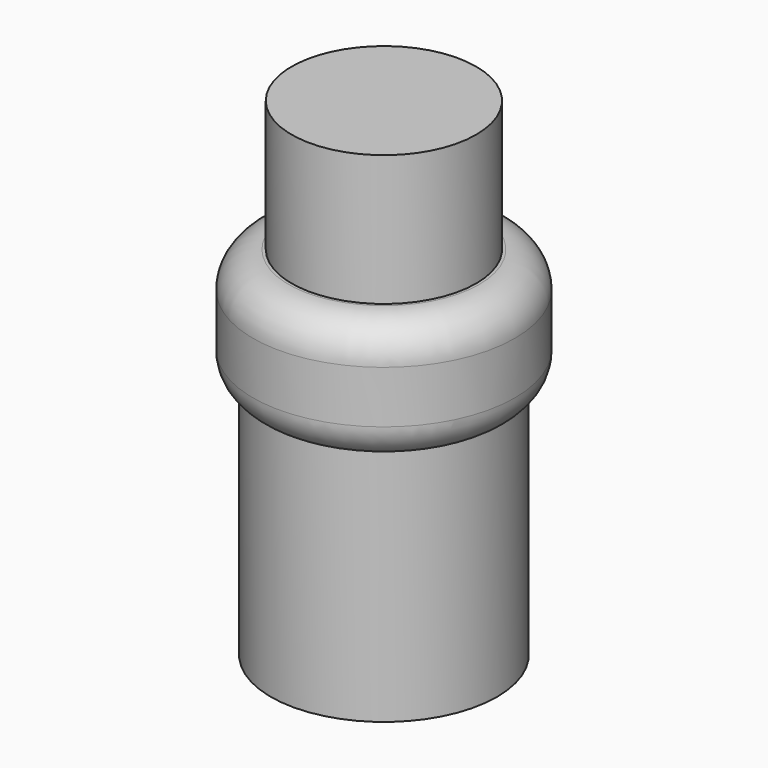
from build123d import *

# Parameters (mm, degrees)
F0_R     = 4.75
F1_DEPTH = 10
F2_R     = 5.5
F3_DEPTH = 5
F4_R     = 3.875
F5_DEPTH = 5.5


# Not quite as in the source:
# - a fillet or chamfer that OpenCascade refuses, or shapes differently, is made with other operations: its cross-section is extruded or revolved along the edge and cut away or added


with BuildPart() as f1:
    # F0 (on Top) → F1 (new body)
    with BuildSketch(Plane.XY):
        Circle(F0_R)
    extrude(amount=F1_DEPTH)

    # F2 (on face) → F3 (join)
    with BuildSketch(Plane.XY.offset(10)):
        Circle(F2_R)
    extrude(amount=F3_DEPTH)

    # F4 (on face) → F5 (join)
    with BuildSketch(Plane.XY.offset(15)):
        Circle(F4_R)
    extrude(amount=F5_DEPTH)

    # F6: fillet of radius 1.5 on 2 edges, made by hand

    # F6_s1 → F6_t2 (revolve, cut)
    with BuildSketch(Plane.XZ):
        with BuildLine():
            ThreePointArc((5.5, 13.5), (5.0606601718, 14.5606601718), (4, 15))
            Line((4, 15), (5.5, 15))
            Line((5.5, 15), (5.5, 13.5))
        make_face()
    revolve(axis=Axis((0, 0, 15), (0, 0, 1)), mode=Mode.SUBTRACT)

    # F6_s3 → F6_t4 (revolve, cut)
    with BuildSketch(Plane.XZ):
        with BuildLine():
            ThreePointArc((5.5, 11.2990381057), (5.2990381057, 10.5490381057), (4.75, 10))
            Line((4.75, 10), (5.5, 10))
            Line((5.5, 10), (5.5, 11.2990381057))
        make_face()
    revolve(axis=Axis((0, 0, 10), (0, 0, 1)), mode=Mode.SUBTRACT)


solid = f1.part
